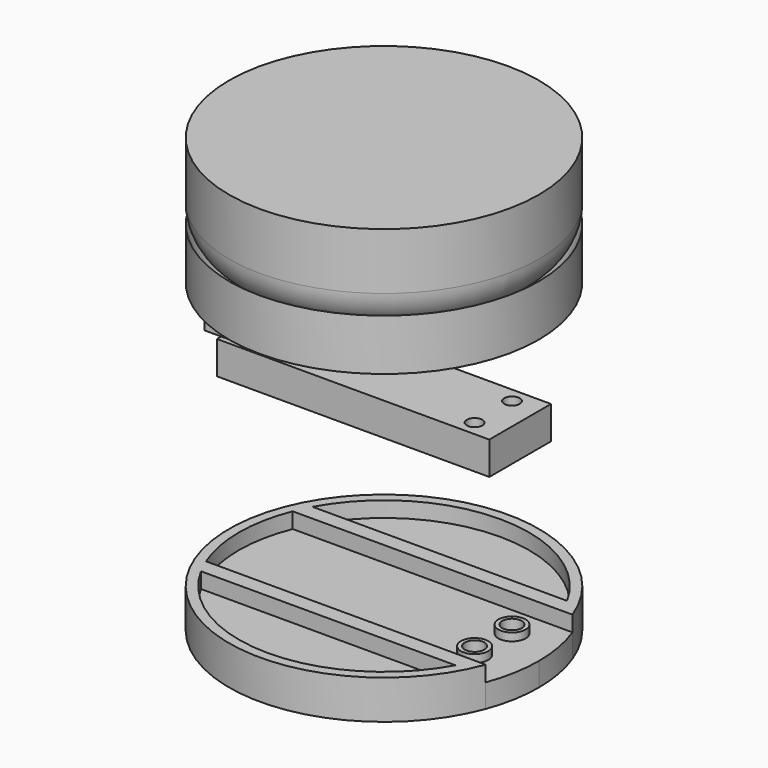
from build123d import *

# Parameters (mm, degrees)
F2_W      = 34.92
F2_H      = 9.89
F2_R      = 1.275
F2_R_2    = 0.9975
F3_DEPTH  = 4.22
F4_DEPTH  = 25
F8_W      = 6.895
F8_H      = 13.89
F8_R      = 1.5675
F9_DEPTH  = 1.1
F11_R     = 1.75
F11_R_2   = 1.25
F12_DEPTH = 3
F13_DEPTH = 4
F14_DEPTH = 5
F6_R      = 2.25
F15_DEPTH = 9.63
F16_R     = 2.875
F17_DEPTH = 1.5


with BuildPart() as f1:
    # F0 (on Front) → F1 (revolve)
    with BuildSketch(Plane.XZ):
        with BuildLine():
            Line((-14.765, 18.2661092722), (-12.945, 18.2661092722))
            Line((-12.945, 18.2661092722), (-10.925, 20.1661092722))
            Line((-10.925, 20.1661092722), (0, 20.1661092722))
            Line((0, 20.1661092722), (0, 30.6185409427))
            Line((0, 30.6185409427), (-19.855, 30.6185409427))
            Line((-19.855, 30.6185409427), (-19.855, 23.3561092722))
            ThreePointArc((-19.855, 23.3561092722), (-18.3641735162, 19.756935756), (-14.765, 18.2661092722))
        make_face()
    revolve(axis=Axis((0, 0, 17.6021158695), (0, 0, 1)))


with BuildPart() as f1b:
    # F0 (on Front) → F1, piece 2 (revolve)
    with BuildSketch(Plane.XZ):
        with BuildLine():
            Line((-10.5286014899, 19.1661091083), (-12.5486014899, 17.2661091083))
            Line((-12.5486014899, 17.2661091083), (-14.9934996444, 17.2661091083))
            ThreePointArc((-14.9934996444, 17.2661091083), (-18.0128234644, 18.2583312142), (-19.855, 20.848158747))
            Line((-19.855, 20.848158747), (-19.855, 14.2661091083))
            Line((-19.855, 14.2661091083), (0, 14.2661091083))
            Line((0, 14.2661091083), (0, 19.1661091083))
            Line((0, 19.1661091083), (-10.5286014899, 19.1661091083))
        make_face()
    revolve(axis=Axis((0, 0, 17.6021158695), (0, 0, 1)))

    # F2 (on Top) → F4 (cut)
    with BuildSketch(Plane.XY):
        with Locations((-14.0125, -2.9975)):
            Circle(F2_R)
        with Locations((-14.0125, -2.9975)):
            Circle(F2_R_2, mode=Mode.SUBTRACT)
        with Locations((-14.0125, 2.9975)):
            Circle(F2_R)
        with Locations((-14.0125, 2.9975)):
            Circle(F2_R_2, mode=Mode.SUBTRACT)
        with Locations((-14.0125, -2.9975)):
            Circle(F2_R_2)
        with Locations((-14.0125, 2.9975)):
            Circle(F2_R_2)
    extrude(amount=F4_DEPTH, mode=Mode.SUBTRACT)

    # F6 (on offset) → F15 (cut)
    with BuildSketch(Plane.XY.offset(25)):
        with Locations((-14.0125, 2.9975)):
            Circle(F6_R)
        with Locations((-14.0125, -2.9975)):
            Circle(F6_R)
    extrude(amount=-F15_DEPTH, mode=Mode.SUBTRACT)


with BuildPart() as f3:
    # F2 (on Top) → F3 (new body)
    with BuildSketch(Plane.XY):
        Rectangle(F2_W, F2_H)
        with Locations((-14.0125, -2.9975)):
            Circle(F2_R, mode=Mode.SUBTRACT)
        with Locations((14.0125, -2.9975)):
            Circle(F2_R, mode=Mode.SUBTRACT)
        with Locations((-14.0125, 2.9975)):
            Circle(F2_R, mode=Mode.SUBTRACT)
        with Locations((14.0125, 2.9975)):
            Circle(F2_R, mode=Mode.SUBTRACT)
        with Locations((-14.0125, 2.9975)):
            Circle(F2_R)
        with Locations((-14.0125, 2.9975)):
            Circle(F2_R_2, mode=Mode.SUBTRACT)
        with Locations((-14.0125, -2.9975)):
            Circle(F2_R)
        with Locations((-14.0125, -2.9975)):
            Circle(F2_R_2, mode=Mode.SUBTRACT)
        with Locations((14.0125, 2.9975)):
            Circle(F2_R)
        with Locations((14.0125, 2.9975)):
            Circle(F2_R_2, mode=Mode.SUBTRACT)
        with Locations((14.0125, -2.9975)):
            Circle(F2_R)
        with Locations((14.0125, -2.9975)):
            Circle(F2_R_2, mode=Mode.SUBTRACT)
    extrude(amount=F3_DEPTH)


with BuildPart() as f9:
    # F8 (on offset) → F9 (new body)
    with BuildSketch(Plane.XY.offset(6)):
        with Locations((-14.0125, 0)):
            Rectangle(F8_W, F8_H)
        with Locations((-14.0125, -3.0175)):
            Circle(F8_R, mode=Mode.SUBTRACT)
        with Locations((-14.0125, 3.0175)):
            Circle(F8_R, mode=Mode.SUBTRACT)
    extrude(amount=F9_DEPTH)


with BuildPart() as f12:
    # F11 (on offset) → F12 (new body)
    with BuildSketch(Plane.XY.offset(-25)):
        with BuildLine():
            ThreePointArc((18.6007526729, -6.945), (19.5389223004, -3.52867402), (19.855, 0))
            ThreePointArc((19.855, 0), (19.5389223004, 3.52867402), (18.6007526729, 6.945))
            Line((18.6007526729, 6.945), (17.2601564303, 6.945))
            ThreePointArc((17.2601564303, 6.945), (18.2656951057, 3.5370054151), (18.605, 0))
            ThreePointArc((18.605, 0), (18.2656951057, -3.5370054151), (17.2601564303, -6.945))
            Line((17.2601564303, -6.945), (18.6007526729, -6.945))
        make_face()
        with BuildLine():
            Line((17.2601564303, 6.945), (18.6007526729, 6.945))
            ThreePointArc((18.6007526729, 6.945), (-19.855, 0), (18.6007526729, -6.945))
            Line((18.6007526729, -6.945), (17.2601564303, -6.945))
            ThreePointArc((17.2601564303, -6.945), (16.81662867, -7.9590844432), (16.3135832974, -8.945))
            ThreePointArc((16.3135832974, -8.945), (0, -18.605), (-16.3135832974, -8.945))
            ThreePointArc((-16.3135832974, -8.945), (-16.81662867, -7.9590844432), (-17.2601564303, -6.945))
            ThreePointArc((-17.2601564303, -6.945), (-18.605, 0), (-17.2601564303, 6.945))
            ThreePointArc((-17.2601564303, 6.945), (-16.81662867, 7.9590844432), (-16.3135832974, 8.945))
            ThreePointArc((-16.3135832974, 8.945), (0, 18.605), (16.3135832974, 8.945))
            ThreePointArc((16.3135832974, 8.945), (16.81662867, 7.9590844432), (17.2601564303, 6.945))
        make_face()
        with BuildLine():
            ThreePointArc((-16.3135832974, -8.945), (0, -18.605), (16.3135832974, -8.945))
            Line((16.3135832974, -8.945), (-16.3135832974, -8.945))
        make_face()
        with BuildLine():
            ThreePointArc((16.3135832974, -8.945), (16.81662867, -7.9590844432), (17.2601564303, -6.945))
            Line((17.2601564303, -6.945), (-17.2601564303, -6.945))
            ThreePointArc((-17.2601564303, -6.945), (-16.81662867, -7.9590844432), (-16.3135832974, -8.945))
            Line((-16.3135832974, -8.945), (16.3135832974, -8.945))
        make_face()
        with BuildLine():
            ThreePointArc((18.605, 0), (18.2656951057, 3.5370054151), (17.2601564303, 6.945))
            Line((17.2601564303, 6.945), (-17.2601564303, 6.945))
            ThreePointArc((-17.2601564303, 6.945), (-18.605, 0), (-17.2601564303, -6.945))
            Line((-17.2601564303, -6.945), (17.2601564303, -6.945))
            ThreePointArc((17.2601564303, -6.945), (18.2656951057, -3.5370054151), (18.605, 0))
        make_face()
        with Locations((14.0125, -2.9975)):
            Circle(F11_R, mode=Mode.SUBTRACT)
        with Locations((14.0125, 2.9975)):
            Circle(F11_R, mode=Mode.SUBTRACT)
        with BuildLine():
            Line((-17.2601564303, 6.945), (17.2601564303, 6.945))
            ThreePointArc((17.2601564303, 6.945), (16.81662867, 7.9590844432), (16.3135832974, 8.945))
            Line((16.3135832974, 8.945), (-16.3135832974, 8.945))
            ThreePointArc((-16.3135832974, 8.945), (-16.81662867, 7.9590844432), (-17.2601564303, 6.945))
        make_face()
        with BuildLine():
            Line((-16.3135832974, 8.945), (16.3135832974, 8.945))
            ThreePointArc((16.3135832974, 8.945), (0, 18.605), (-16.3135832974, 8.945))
        make_face()
        with Locations((14.0125, -2.9975)):
            Circle(F11_R)
        with Locations((14.0125, -2.9975)):
            Circle(F11_R_2, mode=Mode.SUBTRACT)
        with Locations((14.0125, 2.9975)):
            Circle(F11_R)
        with Locations((14.0125, 2.9975)):
            Circle(F11_R_2, mode=Mode.SUBTRACT)
    extrude(amount=F12_DEPTH)

    # F11 (on offset) → F13 (join)
    with BuildSketch(Plane.XY.offset(-25)):
        with Locations((14.0125, -2.9975)):
            Circle(F11_R)
        with Locations((14.0125, -2.9975)):
            Circle(F11_R_2, mode=Mode.SUBTRACT)
        with Locations((14.0125, 2.9975)):
            Circle(F11_R)
        with Locations((14.0125, 2.9975)):
            Circle(F11_R_2, mode=Mode.SUBTRACT)
    extrude(amount=F13_DEPTH)

    # F11 (on offset) → F14 (join)
    with BuildSketch(Plane.XY.offset(-25)):
        with BuildLine():
            ThreePointArc((16.3135832974, -8.945), (16.81662867, -7.9590844432), (17.2601564303, -6.945))
            Line((17.2601564303, -6.945), (-17.2601564303, -6.945))
            ThreePointArc((-17.2601564303, -6.945), (-16.81662867, -7.9590844432), (-16.3135832974, -8.945))
            Line((-16.3135832974, -8.945), (16.3135832974, -8.945))
        make_face()
        with BuildLine():
            Line((17.2601564303, 6.945), (18.6007526729, 6.945))
            ThreePointArc((18.6007526729, 6.945), (-19.855, 0), (18.6007526729, -6.945))
            Line((18.6007526729, -6.945), (17.2601564303, -6.945))
            ThreePointArc((17.2601564303, -6.945), (16.81662867, -7.9590844432), (16.3135832974, -8.945))
            ThreePointArc((16.3135832974, -8.945), (0, -18.605), (-16.3135832974, -8.945))
            ThreePointArc((-16.3135832974, -8.945), (-16.81662867, -7.9590844432), (-17.2601564303, -6.945))
            ThreePointArc((-17.2601564303, -6.945), (-18.605, 0), (-17.2601564303, 6.945))
            ThreePointArc((-17.2601564303, 6.945), (-16.81662867, 7.9590844432), (-16.3135832974, 8.945))
            ThreePointArc((-16.3135832974, 8.945), (0, 18.605), (16.3135832974, 8.945))
            ThreePointArc((16.3135832974, 8.945), (16.81662867, 7.9590844432), (17.2601564303, 6.945))
        make_face()
        with BuildLine():
            Line((-17.2601564303, 6.945), (17.2601564303, 6.945))
            ThreePointArc((17.2601564303, 6.945), (16.81662867, 7.9590844432), (16.3135832974, 8.945))
            Line((16.3135832974, 8.945), (-16.3135832974, 8.945))
            ThreePointArc((-16.3135832974, 8.945), (-16.81662867, 7.9590844432), (-17.2601564303, 6.945))
        make_face()
    extrude(amount=F14_DEPTH)

    # F16 (on offset) → F17 (cut)
    with BuildSketch(Plane.XY.offset(-25)):
        with Locations((14.0125, -2.9975)):
            Circle(F16_R)
        with Locations((14.0125, 2.9975)):
            Circle(F16_R)
    extrude(amount=F17_DEPTH, mode=Mode.SUBTRACT)


solid = Compound([f1.part, f1b.part, f3.part, f9.part, f12.part])
